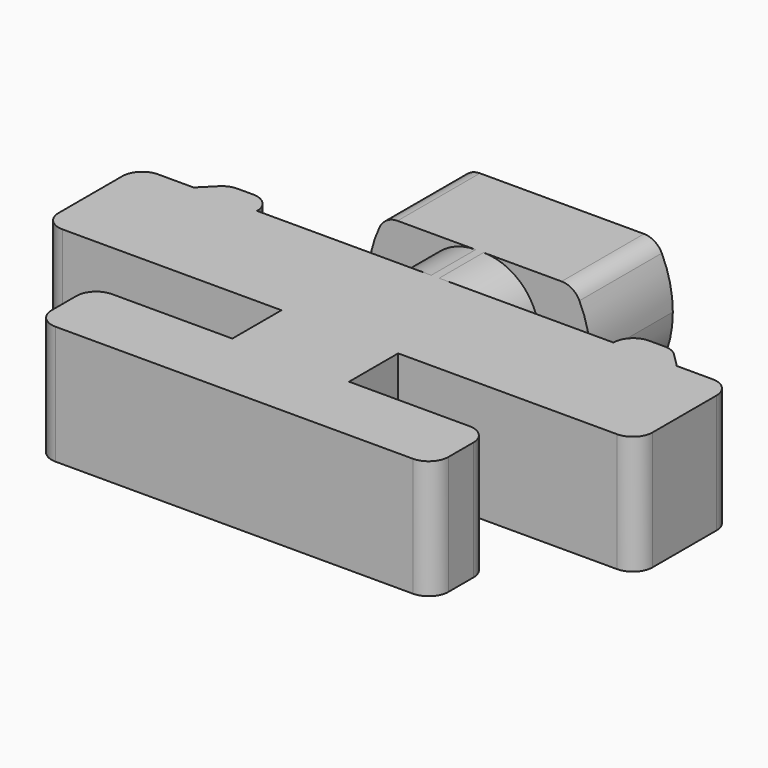
from build123d import *

# Parameters (mm, degrees)
F2_DEPTH = 3
F4_DEPTH = 2.6
F5_R     = 0.49999
F6_R     = 1.4


# Not quite as in the source:
# - a fillet or chamfer is up to 0.001 mm smaller than in the source, because OpenCascade refuses the exact size


with BuildPart() as f2:
    # F1 (on Top) → F2 (new body)
    with BuildSketch(Plane.XY):
        Polygon((2.8, 1.4), (2.8, 4), (-2.8, 4), (-2.8, 1.4), (-1.5, 1.4), (-1.5, 0), (-4.5, 0), (-4.5, 0.5), (-5.6, 0.5), (-6.1, 0), (-7.5, 0), (-7.5, -3.0118150752), (-1.4735722734, -3.0118150752), (-1.4735722734, -4.5618148234), (-5.01158851, -4.5618148234), (-5.01158851, -6.3443139292), (5.01158851, -6.3443139292), (5.01158851, -4.5618148234), (1.4735722734, -4.5618148234), (1.4735722734, -3.0118150752), (7.5, -3.0118150752), (7.5, 0), (6.1, 0), (5.6, 0.5), (4.5, 0.5), (4.5, 0), (1.5, 0), (1.5, 1.4), align=None)
    extrude(amount=F2_DEPTH)

    # F3 (on face) → F4 (cut, through all)
    with BuildSketch(Plane(origin=(0, 4, 0), x_dir=(-1, 0, 0), z_dir=(0, 1, 0))):
        with BuildLine():
            Line((2.8, 0), (2.8, 1.5))
            ThreePointArc((2.8, 1.5), (2.6888743587, 0.7190040441), (2.3643180835, 0))
            Line((2.3643180835, 0), (2.8, 0))
        make_face()
        with BuildLine():
            ThreePointArc((2.3643180835, 3), (2.6888743587, 2.2809959559), (2.8, 1.5))
            Line((2.8, 1.5), (2.8, 3))
            Line((2.8, 3), (2.3643180835, 3))
        make_face()
        with BuildLine():
            ThreePointArc((-2.3643180835, 0), (0, -1.3), (2.3643180835, 0))
            Line((2.3643180835, 0), (-2.3643180835, 0))
        make_face()
        with BuildLine():
            ThreePointArc((-2.8, 1.5), (-2.6888743587, 2.2809959559), (-2.3643180835, 3))
            Line((-2.3643180835, 3), (-2.8, 3))
            Line((-2.8, 3), (-2.8, 1.5))
        make_face()
        with BuildLine():
            Line((-2.8, 0), (-2.3643180835, 0))
            ThreePointArc((-2.3643180835, 0), (-2.6888743587, 0.7190040441), (-2.8, 1.5))
            Line((-2.8, 1.5), (-2.8, 0))
        make_face()
    extrude(amount=-F4_DEPTH, mode=Mode.SUBTRACT)

    # F5 (radius 0.5 in the source; OpenCascade refuses exactly that, so slightly less here)
    f5_edges = [f2.edges().sort_by_distance(p)[0] for p in [
        (4.5, 0.5, 1.5),
        (5.6, 0.5, 1.5),
        (7.5, 0, 1.5),
        (7.5, -3.011815, 1.5),
        (5.011589, -4.561815, 1.5),
        (5.011589, -6.344314, 1.5),
        (-4.5, 0.5, 1.5),
        (-5.6, 0.5, 1.5),
        (-7.5, 0, 1.5),
        (-7.5, -3.011815, 1.5),
        (-5.011589, -6.344314, 1.5),
        (-5.011589, -4.561815, 1.5),
        (2.364318, 2.7, 3),
        (-2.364318, 2.7, 3),
        (2.364318, 2.7, 0),
        (-2.364318, 2.7, 0),
    ]]
    fillet(f5_edges, radius=F5_R)

    # F6
    f6_edges = [f2.edges().sort_by_distance(p)[0] for p in [
        (1.5, 0.7, 3),
        (-1.5, 0.7, 3),
        (1.5, 0.7, 0),
        (-1.5, 0.7, 0),
    ]]
    fillet(f6_edges, radius=F6_R)


solid = f2.part
